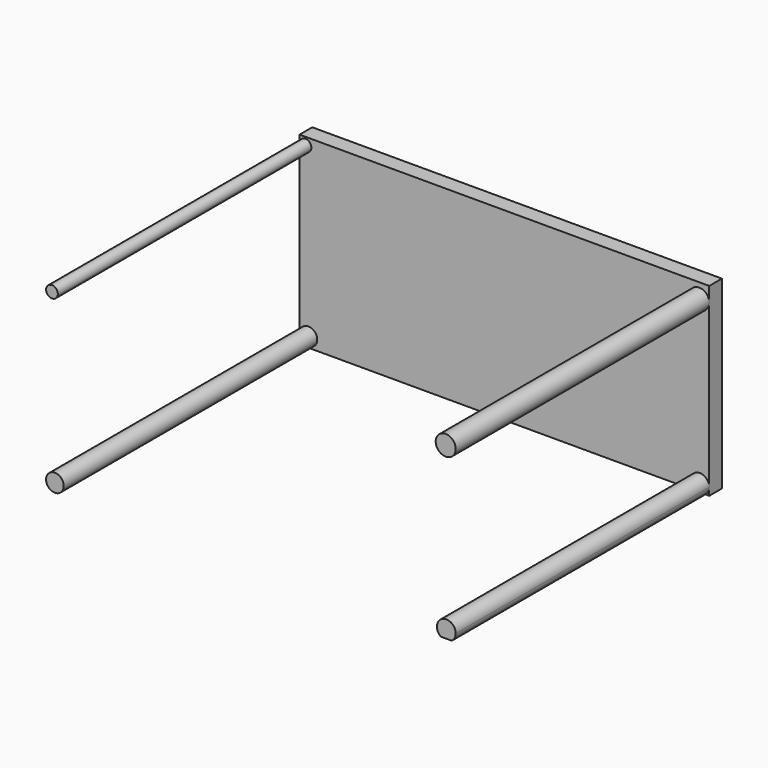
from build123d import *

# Parameters (mm, degrees)
F0_W     = 131.3371732831
F0_H     = 59.2526914552
F1_DEPTH = 5.08
F3_DEPTH = 101.6
F2_R     = 3.2079517841


with BuildPart() as f1:
    # F0 (on Front) → F1 (new body)
    with BuildSketch(Plane.XZ):
        with Locations((5.0949789584, 24.908774998)):
            Rectangle(F0_W, F0_H)
    extrude(amount=F1_DEPTH)

    # F2 (on face) → F3, piece 4 (join)
    with BuildSketch(Plane.XZ.offset(5.08)):
        with BuildLine():
            ThreePointArc((70.7635655999, -2.2644340061), (66.3656159776, 0.4216413008), (65.9842222944, -4.7175707296))
            Line((65.9842222944, -4.7175707296), (69.5044219479, -4.7175707296))
            ThreePointArc((69.5044219479, -4.7175707296), (70.430397428, -3.6431401496), (70.7635655999, -2.2644340061))
        make_face()
    extrude(amount=F3_DEPTH)


with BuildPart() as f3:
    # F2 (on face) → F3 (new body)
    with BuildSketch(Plane.XZ.offset(5.08)):
        with BuildLine():
            ThreePointArc((-60.5736076832, 52.0819835365), (-58.6865805089, 50.1949563622), (-56.7995533347, 52.0819835365))
            ThreePointArc((-56.7995533347, 52.0819835365), (-58.6865805089, 53.9690107107), (-60.5736076832, 52.0819835365))
        make_face()
    extrude(amount=F3_DEPTH)


with BuildPart() as f3b:
    # F2 (on face) → F3, piece 2 (new body)
    with BuildSketch(Plane.XZ.offset(5.08)):
        with BuildLine():
            ThreePointArc((-54.9125224352, -1.5096226707), (-57.7430650433, 1.3209199533), (-60.5736076832, -1.509622639))
            ThreePointArc((-60.5736076832, -1.509622639), (-57.7430650751, -4.3401652947), (-54.9125224352, -1.5096226707))
        make_face()
    extrude(amount=F3_DEPTH)


with BuildPart() as f3c:
    # F2 (on face) → F3, piece 3 (new body)
    with BuildSketch(Plane.XZ.offset(5.08)):
        with Locations((67.5556138158, 49.8175472021)):
            Circle(F2_R)
    extrude(amount=F3_DEPTH)


solid = Compound([f1.part, f3.part, f3b.part, f3c.part])
